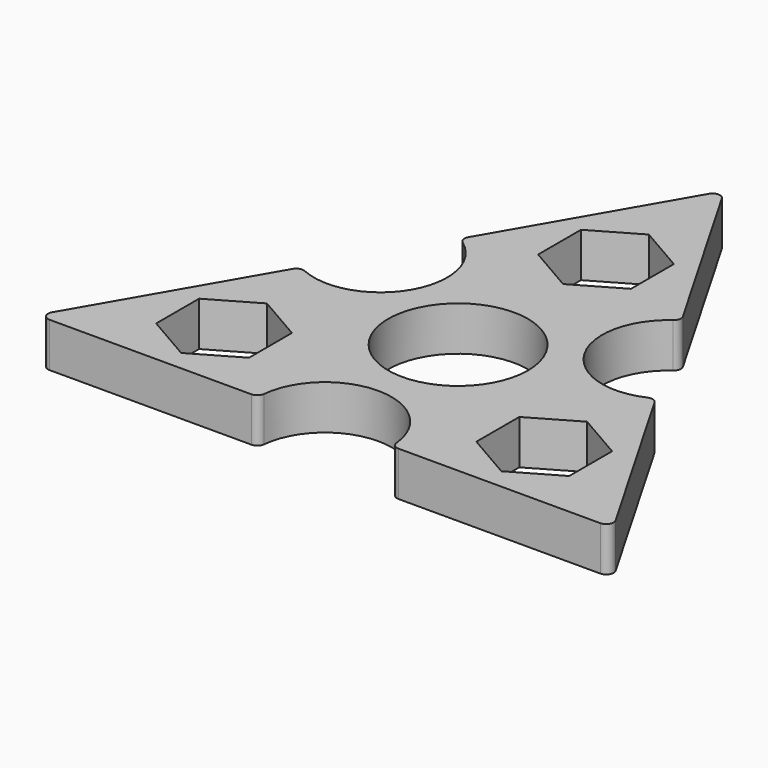
from build123d import *

# Parameters (mm, degrees)
F0_R     = 9.45
F1_DEPTH = 6
F2_R     = 1
F3_R     = 1


with BuildPart() as f1:
    # F0 (on Top) → F1 (new body)
    with BuildSketch(Plane.XY):
        with BuildLine():
            Line((14.9855715851, 19.0442286341), (0, 45))
            Line((0, 45), (-14.9855715851, 19.0442286341))
            ThreePointArc((-14.9855715851, 19.0442286341), (-11.6913429511, 6.75), (-23.9855715851, 3.4557713659))
            Line((-23.9855715851, 3.4557713659), (-38.9711431703, -22.5))
            Line((-38.9711431703, -22.5), (-9, -22.5))
            ThreePointArc((-9, -22.5), (0, -13.5), (9, -22.5))
            Line((9, -22.5), (38.9711431703, -22.5))
            Line((38.9711431703, -22.5), (23.9855715851, 3.4557713659))
            ThreePointArc((23.9855715851, 3.4557713659), (11.6913429511, 6.75), (14.9855715851, 19.0442286341))
        make_face()
        Polygon((-15.3719509172, -16.125), (-21.6506350946, -19.75), (-27.929319272, -16.125), (-27.929319272, -8.875), (-21.6506350946, -5.25), (-15.3719509172, -8.875), align=None, mode=Mode.SUBTRACT)
        Polygon((21.6506350946, -5.25), (27.929319272, -8.875), (27.929319272, -16.125), (21.6506350946, -19.75), (15.3719509172, -16.125), (15.3719509172, -8.875), align=None, mode=Mode.SUBTRACT)
        Circle(F0_R, mode=Mode.SUBTRACT)
        Polygon((-6.2786841774, 28.625), (0, 32.25), (6.2786841774, 28.625), (6.2786841774, 21.375), (0, 17.75), (-6.2786841774, 21.375), align=None, mode=Mode.SUBTRACT)
    extrude(amount=F1_DEPTH)

    # F2
    f2_edges = [f1.edges().sort_by_distance(p)[0] for p in [
        (14.985572, 19.044229, 3),
        (-23.985572, 3.455771, 3),
        (9, -22.5, 3),
    ]]
    fillet(f2_edges, radius=F2_R)

    # F3
    f3_edges = [f1.edges().sort_by_distance(p)[0] for p in [
        (0, 45, 3),
        (38.971143, -22.5, 3),
        (-38.971143, -22.5, 3),
        (-14.985572, 19.044229, 3),
        (23.985572, 3.455771, 3),
        (-9, -22.5, 3),
    ]]
    fillet(f3_edges, radius=F3_R)


solid = f1.part
